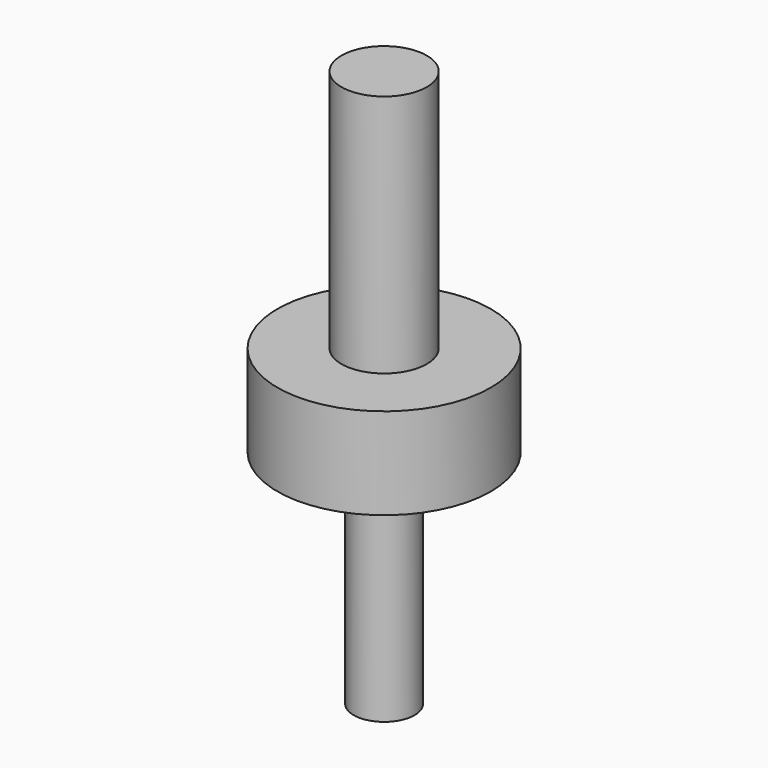
from build123d import *

# Parameters (mm, degrees)
F0_R     = 5.55625
F1_DEPTH = 4.7625
F2_R     = 2.2225
F3_DEPTH = 12.7
F4_R     = 1.5875
F5_DEPTH = 11.5443


# Not quite as in the source:
# - a length typed as a fraction of an inch, garbled in the dataset ("3 / 203.2 mm" for 3/8 in), is restored


with BuildPart() as f1:
    # F0 (on Top) → F1 (new body)
    with BuildSketch(Plane.XY):
        Circle(F0_R)
    extrude(amount=F1_DEPTH)

    # F2 (on face) → F3 (join)
    with BuildSketch(Plane.XY.offset(4.7625)):
        Circle(F2_R)
    extrude(amount=F3_DEPTH)

    # F4 (on face) → F5 (join)
    with BuildSketch(Plane(origin=(0, 0, 0), x_dir=(1, 0, 0), z_dir=(0, 0, -1))):
        Circle(F4_R)
    extrude(amount=F5_DEPTH)


solid = f1.part
